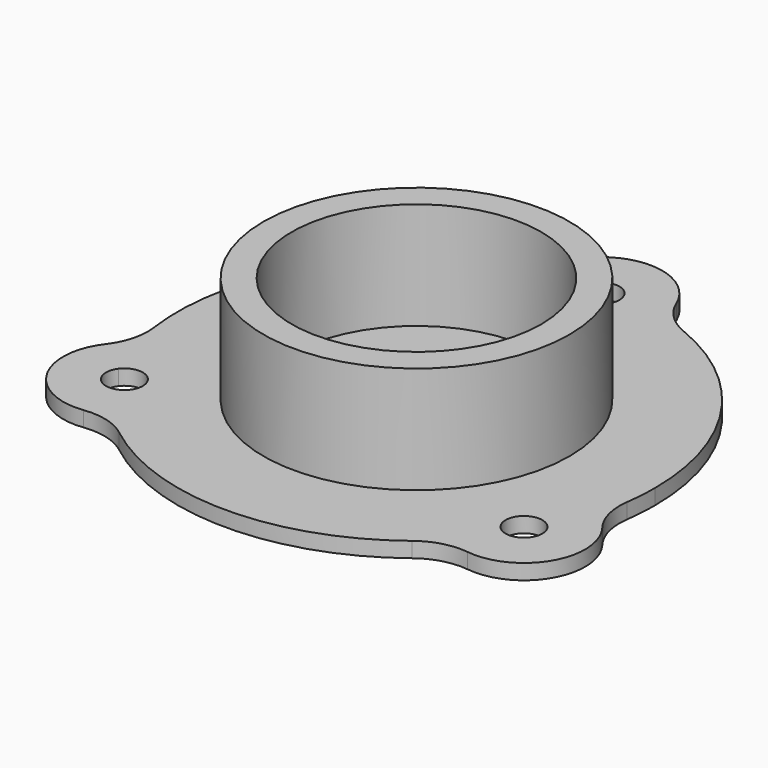
from build123d import *

# Parameters (mm, degrees)
F0_R     = 15.875
F0_R_2   = 12.954
F1_DEPTH = 12.7
F0_W     = 8.89
F0_H     = 8.89
F2_DEPTH = 1.5875
F3_DEPTH = 1.5875
F4_R     = 6.35


with BuildPart() as f1:
    # F0 (on Top) → F1 (new body)
    with BuildSketch(Plane.XY):
        Circle(F0_R)
        Circle(F0_R_2, mode=Mode.SUBTRACT)
    extrude(amount=F1_DEPTH)

    # F0 (on Top) → F2 (join)
    with BuildSketch(Plane.XY):
        Circle(F0_R_2)
        Rectangle(F0_W, F0_H, mode=Mode.SUBTRACT)
    extrude(amount=F2_DEPTH)

    # F0 (on Top) → F3 (join)
    with BuildSketch(Plane.XY):
        with BuildLine():
            ThreePointArc((23.9050999455, -6.4692674698), (24.5490837421, -3.2630832697), (24.765, 0))
            ThreePointArc((24.765, 0), (19.6285885254, 15.1004548773), (6.35, 23.9370575677))
            ThreePointArc((6.35, 23.9370575677), (4.0651088886, 24.4290833787), (1.7440091422, 24.703515076))
            ThreePointArc((1.7440091422, 24.703515076), (1.8643178935, 24.3286489263), (1.905, 23.9370575677))
            ThreePointArc((1.905, 23.9370575677), (-0.3915913586, 22.0727396742), (-1.7440091422, 24.703515076))
            ThreePointArc((-1.7440091422, 24.703515076), (-4.0651088886, 24.4290833787), (-6.35, 23.9370575677))
            ThreePointArc((-6.35, 23.9370575677), (-21.4471191247, 12.3825), (-23.9050999455, -6.4692674698))
            ThreePointArc((-23.9050999455, -6.4692674698), (-23.1887612414, -8.6940541227), (-22.2658761897, -10.8414013165))
            ThreePointArc((-22.2658761897, -10.8414013165), (-20.1370690632, -10.1581864481), (-18.8250999455, -11.9685287839))
            ThreePointArc((-18.8250999455, -11.9685287839), (-19.3113489683, -13.239815795), (-20.5218670475, -13.8621137596))
            ThreePointArc((-20.5218670475, -13.8621137596), (-19.1236523528, -15.735029256), (-17.5550999455, -17.4677900979))
            ThreePointArc((-17.5550999455, -17.4677900979), (0, -24.765), (17.5550999455, -17.4677900979))
            ThreePointArc((17.5550999455, -17.4677900979), (19.1236523528, -15.735029256), (20.5218670475, -13.8621137596))
            ThreePointArc((20.5218670475, -13.8621137596), (19.0803215513, -11.0160287839), (22.2658761897, -10.8414013165))
            ThreePointArc((22.2658761897, -10.8414013165), (23.1887612414, -8.6940541227), (23.9050999455, -6.4692674698))
        make_face()
        Circle(F0_R, mode=Mode.SUBTRACT)
        with BuildLine():
            ThreePointArc((1.7440091422, 24.703515076), (4.0651088886, 24.4290833787), (6.35, 23.9370575677))
            ThreePointArc((6.35, 23.9370575677), (0, 30.2870575677), (-6.35, 23.9370575677))
            ThreePointArc((-6.35, 23.9370575677), (-4.0651088886, 24.4290833787), (-1.7440091422, 24.703515076))
            ThreePointArc((-1.7440091422, 24.703515076), (0, 25.8420575677), (1.7440091422, 24.703515076))
        make_face()
        with BuildLine():
            ThreePointArc((17.5550999455, -17.4677900979), (26.2293612595, -15.1435287839), (23.9050999455, -6.4692674698))
            ThreePointArc((23.9050999455, -6.4692674698), (23.1887612414, -8.6940541227), (22.2658761897, -10.8414013165))
            ThreePointArc((22.2658761897, -10.8414013165), (22.5404422812, -11.3754979015), (22.6350999455, -11.9685287839))
            ThreePointArc((22.6350999455, -11.9685287839), (22.0013869566, -13.3872797611), (20.5218670475, -13.8621137596))
            ThreePointArc((20.5218670475, -13.8621137596), (19.1236523528, -15.735029256), (17.5550999455, -17.4677900979))
        make_face()
        with BuildLine():
            ThreePointArc((-22.2658761897, -10.8414013165), (-23.1887612414, -8.6940541227), (-23.9050999455, -6.4692674698))
            ThreePointArc((-23.9050999455, -6.4692674698), (-26.2293612595, -15.1435287839), (-17.5550999455, -17.4677900979))
            ThreePointArc((-17.5550999455, -17.4677900979), (-19.1236523528, -15.735029256), (-20.5218670475, -13.8621137596))
            ThreePointArc((-20.5218670475, -13.8621137596), (-22.3798783397, -12.9210287839), (-22.2658761897, -10.8414013165))
        make_face()
    extrude(amount=F3_DEPTH)

    # F4
    f4_edges = [f1.edges().sort_by_distance(p)[0] for p in [
        (-23.9051, -6.469267, 0.79375),
        (17.5551, -17.46779, 0.79375),
        (6.35, 23.937058, 0.79375),
        (23.9051, -6.469267, 0.79375),
        (-6.35, 23.937058, 0.79375),
        (-17.5551, -17.46779, 0.79375),
    ]]
    fillet(f4_edges, radius=F4_R)


solid = f1.part
